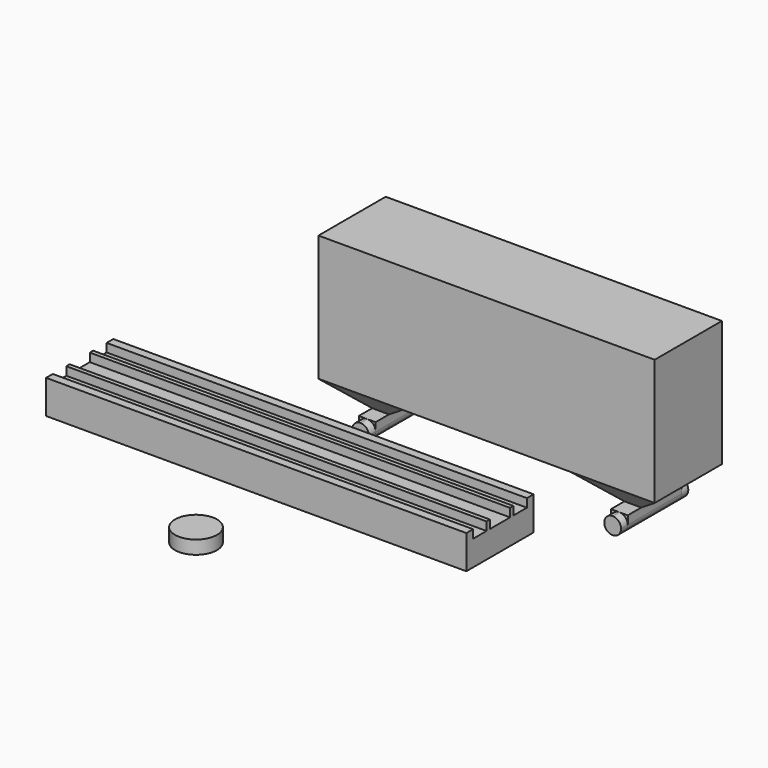
from build123d import *

# Parameters (mm, degrees)
F0_W         = 127
F0_H         = 25.4
F1_DEPTH     = 7.62
F2_W         = 127
F2_H         = 1.27
F2_H_2       = 2.54
F3_DEPTH     = 2.54
F4_W         = 101.6
F4_H         = 25.4
F5_DEPTH     = 38.1
F6_W         = 25.4
F6_H         = 25.4
F8_W         = 5.08
F8_H         = 10.16
F11_DEPTH    = 5.08
F12_T1_DEPTH = 22.86
F13_DEPTH    = 5.08
F14_DEPTH    = 5.08
F17_DEPTH    = 2.54
F20_DEPTH    = 2.54
F21_R        = 6.35
F22_DEPTH    = 4.064
F23_R        = 3.556
F24_DEPTH    = 2.794


# Not quite as in the source:
# - a fillet or chamfer that OpenCascade refuses, or shapes differently, is made with other operations: its cross-section is extruded or revolved along the edge and cut away or added


with BuildPart() as f1:
    # F0 (on Top) → F1 (new body)
    with BuildSketch(Plane.XY):
        with Locations((-4.4709164057, -0.284396112)):
            Rectangle(F0_W, F0_H)
    extrude(amount=F1_DEPTH)

    # F2 (on face) → F3 (join)
    with BuildSketch(Plane.XY.offset(7.62)):
        with Locations((-4.4709164057, 4.160603888)):
            Rectangle(F2_W, F2_H)
        with Locations((-4.4709164057, 11.145603888)):
            Rectangle(F2_W, F2_H_2)
        with Locations((-4.4709164057, -4.729396112)):
            Rectangle(F2_W, F2_H)
        with Locations((-4.4709164057, -11.714396112)):
            Rectangle(F2_W, F2_H_2)
    extrude(amount=F3_DEPTH)


with BuildPart() as f5:
    # F4 (on Top) → F5 (new body)
    with BuildSketch(Plane.XY):
        with Locations((21.1237182349, 54.7262806648)):
            Rectangle(F4_W, F4_H)
    extrude(amount=F5_DEPTH)

    # F6 (on face) → F9 section 0
    with BuildSketch(Plane(origin=(0, 0, 0), x_dir=(1, 0, 0), z_dir=(0, 0, -1))):
        with Locations((-16.9762817651, -54.7262806648)):
            Rectangle(F6_W, F6_H)
    # F8 (on offset) → F9 section 1
    with BuildSketch(Plane.XY.offset(-7.62)):
        with Locations((-16.9762817651, 54.7262806648)):
            Rectangle(F8_W, F8_H)
    loft()

    # F8 (on offset) → F10 section 0
    with BuildSketch(Plane.XY.offset(-7.62)):
        with Locations((59.2237182349, 54.7262806648)):
            Rectangle(F8_W, F8_H)
    # F6 (on face) → F10 section 1
    with BuildSketch(Plane(origin=(0, 0, 0), x_dir=(1, 0, 0), z_dir=(0, 0, -1))):
        with Locations((59.2237182349, -54.7262806648)):
            Rectangle(F6_W, F6_H)
    loft()

    # F11 (add): faces of the model
    f11_faces = [f5.faces().sort_by_distance(p)[0] for p in [
        (59.2237182349, 54.7262806648, -7.62),
        (-16.9762817651, 54.7262806648, -7.62),
    ]]
    extrude(f11_faces, amount=F11_DEPTH)

    # F12: fillet of radius 2.54 on 8 edges, made by hand

    # F12_s2 → F12_t1 (cut)
    with BuildSketch(Plane.XZ.offset(-66.1562806648)):
        with BuildLine():
            ThreePointArc((61.7637182349, -10.16), (61.0197694591, -11.9560512242), (59.2237182349, -12.7))
            Line((59.2237182349, -12.7), (61.7637182349, -12.7))
            Line((61.7637182349, -12.7), (61.7637182349, -10.16))
        make_face()
        with BuildLine():
            ThreePointArc((56.6837182349, -10.16), (57.4276670107, -11.9560512242), (59.2237182349, -12.7))
            Line((59.2237182349, -12.7), (56.6837182349, -12.7))
            Line((56.6837182349, -12.7), (56.6837182349, -10.16))
        make_face()
        with BuildLine():
            ThreePointArc((-19.5162817651, -10.16), (-18.7723329893, -11.9560512242), (-16.9762817651, -12.7))
            Line((-16.9762817651, -12.7), (-19.5162817651, -12.7))
            Line((-19.5162817651, -12.7), (-19.5162817651, -10.16))
        make_face()
        with BuildLine():
            ThreePointArc((-14.4362817651, -10.16), (-15.1802305409, -11.9560512242), (-16.9762817651, -12.7))
            Line((-16.9762817651, -12.7), (-14.4362817651, -12.7))
            Line((-14.4362817651, -12.7), (-14.4362817651, -10.16))
        make_face()
    extrude(amount=F12_T1_DEPTH, mode=Mode.SUBTRACT)

    # F13 (add): faces of the model
    f13_faces = [f5.faces().sort_by_distance(p)[0] for p in [
        (-16.9762817651, 59.8062806648, -9.9228913583),
        (59.2237182349, 59.8062806648, -9.9228913583),
    ]]
    extrude(f13_faces, amount=F13_DEPTH)

    # F14 (add): faces of the model
    f14_faces = [f5.faces().sort_by_distance(p)[0] for p in [
        (-16.9762817651, 49.6462806648, -9.9228913583),
        (59.2237182349, 49.6462806648, -9.9228913583),
    ]]
    extrude(f14_faces, amount=F14_DEPTH)

    # F16 (on face) + F15 (on face) → F17 (join)
    with BuildSketch(Plane(origin=(0, 64.8862806648, 0), x_dir=(-1, 0, 0), z_dir=(0, 1, 0))):
        with BuildLine():
            ThreePointArc((16.9762817651, -7.62), (15.1802305409, -11.9560512242), (19.5162817651, -10.16))
            ThreePointArc((19.5162817651, -10.16), (18.7723329893, -8.3639487758), (16.9762817651, -7.62))
        make_face()
    with BuildSketch(Plane(origin=(0, 64.8862806648, 0), x_dir=(-1, 0, 0), z_dir=(0, 1, 0))):
        with BuildLine():
            ThreePointArc((-59.2237182349, -7.62), (-61.0197694591, -11.9560512242), (-56.6837182349, -10.16))
            ThreePointArc((-56.6837182349, -10.16), (-57.4276670107, -8.3639487758), (-59.2237182349, -7.62))
        make_face()
    extrude(amount=F17_DEPTH)

    # F19 (on face) + F18 (on face) → F20 (join)
    with BuildSketch(Plane.XZ.offset(-44.5662806648)):
        with BuildLine():
            ThreePointArc((59.2237182349, -7.62), (57.4276670107, -11.9560512242), (61.7637182349, -10.16))
            ThreePointArc((61.7637182349, -10.16), (61.0197694591, -8.3639487758), (59.2237182349, -7.62))
        make_face()
    with BuildSketch(Plane.XZ.offset(-44.5662806648)):
        with BuildLine():
            ThreePointArc((-16.9762817651, -7.62), (-18.7723329893, -11.9560512242), (-14.4362817651, -10.16))
            ThreePointArc((-14.4362817651, -10.16), (-15.1802305409, -8.3639487758), (-16.9762817651, -7.62))
        make_face()
    extrude(amount=F20_DEPTH)


with BuildPart() as f22:
    # F21 (on Top) → F22 (new body)
    with BuildSketch(Plane.XY):
        with Locations((0, -41.3258223492)):
            Circle(F21_R)
    extrude(amount=F22_DEPTH)

    # F23 (on face) → F24 (cut)
    with BuildSketch(Plane(origin=(0, 0, 0), x_dir=(1, 0, 0), z_dir=(0, 0, -1))):
        with Locations((0, 41.3258223492)):
            Circle(F23_R)
    extrude(amount=-F24_DEPTH, mode=Mode.SUBTRACT)


solid = Compound([f1.part, f5.part, f22.part])
